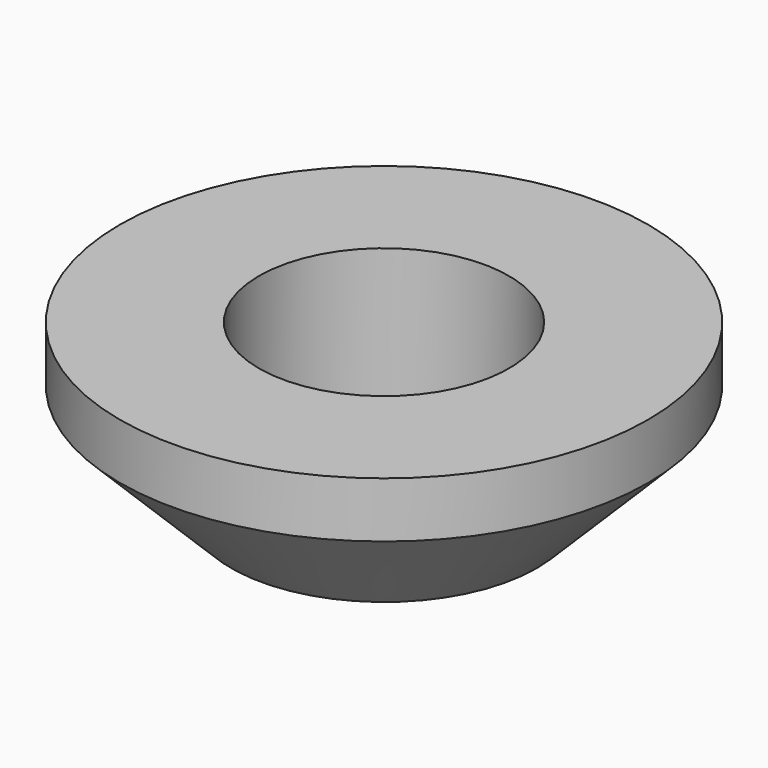
from build123d import *

# Parameters (mm, degrees)
F3_ANGLE = 150
F4_R     = 2.99999
F4_2_R   = 2.99999


# Not quite as in the source:
# - a fillet or chamfer is up to 0.001 mm smaller than in the source, because OpenCascade refuses the exact size


with BuildPart() as f1:
    # F0 (on Front) → F1 (revolve)
    with BuildSketch(Plane.XZ):
        Polygon((-22.5, 0), (-22.5, 30), (-47.5, 30), (-47.5, 20), (-27.5, 0), align=None)
    revolve(axis=Axis((0, 0, 9.4880101401), (0, 0, -1)))


with BuildPart() as f3:
    # F2 (on Front) → F3 (revolve)
    with BuildSketch(Plane.XZ):
        Polygon((-35.2781745931, 14.8492424049), (-39.5208152802, 19.091883092), (-45.1776695297, 13.4350288425), (-40.9350288425, 9.1923881554), align=None)
    revolve(axis=Axis((0, 0, 13.259918429), (0, 0, -1)), revolution_arc=F3_ANGLE)

    # F4 (radius 3 in the source; OpenCascade refuses exactly that, so slightly less here)
    f4_edges = [f3.edges().sort_by_distance(p)[0] for p in [
        (-42.349242, 0, 16.263456),
        (-38.106602, 0, 12.020815),
        (33.001285, 19.053301, 12.020815),
        (36.67552, 21.174621, 16.263456),
    ]]
    fillet(f4_edges, radius=F4_R)


with BuildPart() as f3b:
    # F2 (on Front) → F3, piece 2 (revolve)
    with BuildSketch(Plane.XZ):
        Polygon((-31.7426406871, 11.313708499), (-37.3994949366, 5.6568542495), (-33.1568542495, 1.4142135624), (-27.5, 7.0710678119), align=None)
    revolve(axis=Axis((0, 0, 13.259918429), (0, 0, -1)), revolution_arc=F3_ANGLE)

    # F4#2 (radius 3 in the source; OpenCascade refuses exactly that, so slightly less here)
    f4_2_edges = [f3b.edges().sort_by_distance(p)[0] for p in [
        (-30.328427, 0, 4.242641),
        (-34.571068, 0, 8.485281),
        (26.265188, 15.164214, 4.242641),
        (29.939423, 17.285534, 8.485281),
    ]]
    fillet(f4_2_edges, radius=F4_2_R)


with BuildPart() as f1_1:
    add(f1.part)

    # F5: cut F3b, F3
    add(f3b.part, mode=Mode.SUBTRACT)
    add(f3.part, mode=Mode.SUBTRACT)


solid = f1_1.part
